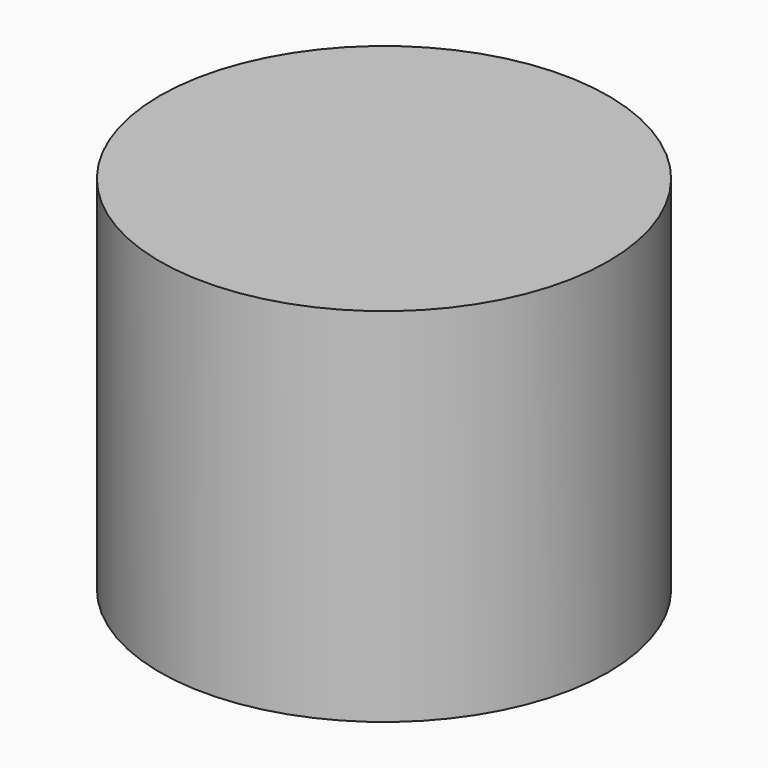
from build123d import *

# Parameters (mm, degrees)
F0_R      = 620
F1_DEPTH  = 994
F2_T      = -6
F3_R      = 620
F4_DEPTH  = 6
F6_R      = 12.5
F7_DEPTH  = 20
F9_R      = 12.5
F10_DEPTH = 20
F12_R     = 12.5
F13_DEPTH = 20
F15_R     = 12.5
F16_DEPTH = 20


with BuildPart() as f1:
    # F0 (on Top) → F1 (new body)
    with BuildSketch(Plane.XY):
        Circle(F0_R)
    extrude(amount=F1_DEPTH)

    # F2
    f2_openings = [f1.faces().sort_by_distance(p)[0] for p in [
        (0, 0, 994),
    ]]
    offset(amount=F2_T, openings=f2_openings)

    # F3 (on face) → F4 (join)
    with BuildSketch(Plane.XY.offset(994)):
        Circle(F3_R)
    extrude(amount=F4_DEPTH)


with BuildPart() as f7:
    # F6 (on offset) → F7 (new body)
    with BuildSketch(Plane.XY.offset(56)):
        with Locations((-443.6559786691, -337.6027585657)):
            Circle(F6_R)
    extrude(amount=F7_DEPTH)


with BuildPart() as f7b:
    # F6 (on offset) → F7, piece 2 (new body)
    with BuildSketch(Plane.XY.offset(56)):
        with Locations((70.5445759711, -553.0187273511)):
            Circle(F6_R)
    extrude(amount=F7_DEPTH)


with BuildPart() as f7c:
    # F6 (on offset) → F7, piece 3 (new body)
    with BuildSketch(Plane.XY.offset(56)):
        with Locations((514.2005546402, -215.4159687854)):
            Circle(F6_R)
    extrude(amount=F7_DEPTH)


with BuildPart() as f7d:
    # F6 (on offset) → F7, piece 4 (new body)
    with BuildSketch(Plane.XY.offset(56)):
        with Locations((443.6559786691, 337.6027585657)):
            Circle(F6_R)
    extrude(amount=F7_DEPTH)


with BuildPart() as f7e:
    # F6 (on offset) → F7, piece 5 (new body)
    with BuildSketch(Plane.XY.offset(56)):
        with Locations((-70.5445759711, 553.0187273511)):
            Circle(F6_R)
    extrude(amount=F7_DEPTH)


with BuildPart() as f7f:
    # F6 (on offset) → F7, piece 6 (new body)
    with BuildSketch(Plane.XY.offset(56)):
        with Locations((-514.2005546402, 215.4159687854)):
            Circle(F6_R)
    extrude(amount=F7_DEPTH)


with BuildPart() as f7g:
    # F6 (on offset) → F7, piece 7 (new body)
    with BuildSketch(Plane.XY.offset(56)):
        Circle(F6_R)
    extrude(amount=F7_DEPTH)


with BuildPart() as f10:
    # F9 (on offset) → F10 (new body)
    with BuildSketch(Plane.XY.offset(256)):
        with Locations((-168.8013792829, 221.8279893345)):
            Circle(F9_R)
    extrude(amount=F10_DEPTH)


with BuildPart() as f10b:
    # F9 (on offset) → F10, piece 2 (new body)
    with BuildSketch(Plane.XY.offset(256)):
        with Locations((-276.5093636756, -35.2722879855)):
            Circle(F9_R)
    extrude(amount=F10_DEPTH)


with BuildPart() as f10c:
    # F9 (on offset) → F10, piece 3 (new body)
    with BuildSketch(Plane.XY.offset(256)):
        with Locations((-107.7079843927, -257.1002773201)):
            Circle(F9_R)
    extrude(amount=F10_DEPTH)


with BuildPart() as f10d:
    # F9 (on offset) → F10, piece 4 (new body)
    with BuildSketch(Plane.XY.offset(256)):
        with Locations((168.8013792829, -221.8279893345)):
            Circle(F9_R)
    extrude(amount=F10_DEPTH)


with BuildPart() as f10e:
    # F9 (on offset) → F10, piece 5 (new body)
    with BuildSketch(Plane.XY.offset(256)):
        with Locations((276.5093636756, 35.2722879855)):
            Circle(F9_R)
    extrude(amount=F10_DEPTH)


with BuildPart() as f10f:
    # F9 (on offset) → F10, piece 6 (new body)
    with BuildSketch(Plane.XY.offset(256)):
        with BuildLine():
            ThreePointArc((120.2079843927, 257.1002773201), (118.1152998658, 264.0239890879), (112.5379388498, 268.629437738))
            ThreePointArc((112.5379388498, 268.629437738), (96.1788239748, 261.9302317772), (102.8780299356, 245.5711169021))
            ThreePointArc((102.8780299356, 245.5711169021), (114.6316961605, 246.692961847), (120.2079843927, 257.1002773201))
        make_face()
    extrude(amount=F10_DEPTH)


with BuildPart() as f13:
    # F12 (on offset) → F13 (new body)
    with BuildSketch(Plane.XY.offset(456)):
        with Locations((-443.6559786691, -337.6027585657)):
            Circle(F12_R)
    extrude(amount=F13_DEPTH)


with BuildPart() as f13b:
    # F12 (on offset) → F13, piece 2 (new body)
    with BuildSketch(Plane.XY.offset(456)):
        with Locations((70.5445759711, -553.0187273511)):
            Circle(F12_R)
    extrude(amount=F13_DEPTH)


with BuildPart() as f13c:
    # F12 (on offset) → F13, piece 3 (new body)
    with BuildSketch(Plane.XY.offset(456)):
        with Locations((514.2005546402, -215.4159687854)):
            Circle(F12_R)
    extrude(amount=F13_DEPTH)


with BuildPart() as f13d:
    # F12 (on offset) → F13, piece 4 (new body)
    with BuildSketch(Plane.XY.offset(456)):
        with Locations((443.6559786691, 337.6027585657)):
            Circle(F12_R)
    extrude(amount=F13_DEPTH)


with BuildPart() as f13e:
    # F12 (on offset) → F13, piece 5 (new body)
    with BuildSketch(Plane.XY.offset(456)):
        with Locations((-70.5445759711, 553.0187273511)):
            Circle(F12_R)
    extrude(amount=F13_DEPTH)


with BuildPart() as f13f:
    # F12 (on offset) → F13, piece 6 (new body)
    with BuildSketch(Plane.XY.offset(456)):
        with Locations((-514.2005546402, 215.4159687854)):
            Circle(F12_R)
    extrude(amount=F13_DEPTH)


with BuildPart() as f13g:
    # F12 (on offset) → F13, piece 7 (new body)
    with BuildSketch(Plane.XY.offset(456)):
        Circle(F12_R)
    extrude(amount=F13_DEPTH)


with BuildPart() as f16:
    # F15 (on offset) → F16 (new body)
    with BuildSketch(Plane.XY.offset(656)):
        with Locations((-168.8013792829, 221.8279893345)):
            Circle(F15_R)
    extrude(amount=F16_DEPTH)


with BuildPart() as f16b:
    # F15 (on offset) → F16, piece 2 (new body)
    with BuildSketch(Plane.XY.offset(656)):
        with BuildLine():
            ThreePointArc((120.2079843927, 257.1002773201), (118.1152998658, 264.0239890879), (112.5379388498, 268.629437738))
            ThreePointArc((112.5379388498, 268.629437738), (96.1788239748, 261.9302317772), (102.8780299356, 245.5711169021))
            ThreePointArc((102.8780299356, 245.5711169021), (114.6316961605, 246.692961847), (120.2079843927, 257.1002773201))
        make_face()
    extrude(amount=F16_DEPTH)


with BuildPart() as f16c:
    # F15 (on offset) → F16, piece 3 (new body)
    with BuildSketch(Plane.XY.offset(656)):
        with Locations((276.5093636756, 35.2722879855)):
            Circle(F15_R)
    extrude(amount=F16_DEPTH)


with BuildPart() as f16d:
    # F15 (on offset) → F16, piece 4 (new body)
    with BuildSketch(Plane.XY.offset(656)):
        with Locations((168.8013792829, -221.8279893345)):
            Circle(F15_R)
    extrude(amount=F16_DEPTH)


with BuildPart() as f16e:
    # F15 (on offset) → F16, piece 5 (new body)
    with BuildSketch(Plane.XY.offset(656)):
        with Locations((-107.7079843927, -257.1002773201)):
            Circle(F15_R)
    extrude(amount=F16_DEPTH)


with BuildPart() as f16f:
    # F15 (on offset) → F16, piece 6 (new body)
    with BuildSketch(Plane.XY.offset(656)):
        with Locations((-276.5093636756, -35.2722879855)):
            Circle(F15_R)
    extrude(amount=F16_DEPTH)


solid = Compound([f1.part, f7.part, f7b.part, f7c.part, f7d.part, f7e.part, f7f.part, f7g.part, f10.part, f10b.part, f10c.part, f10d.part, f10e.part, f10f.part, f13.part, f13b.part, f13c.part, f13d.part, f13e.part, f13f.part, f13g.part, f16.part, f16b.part, f16c.part, f16d.part, f16e.part, f16f.part])
